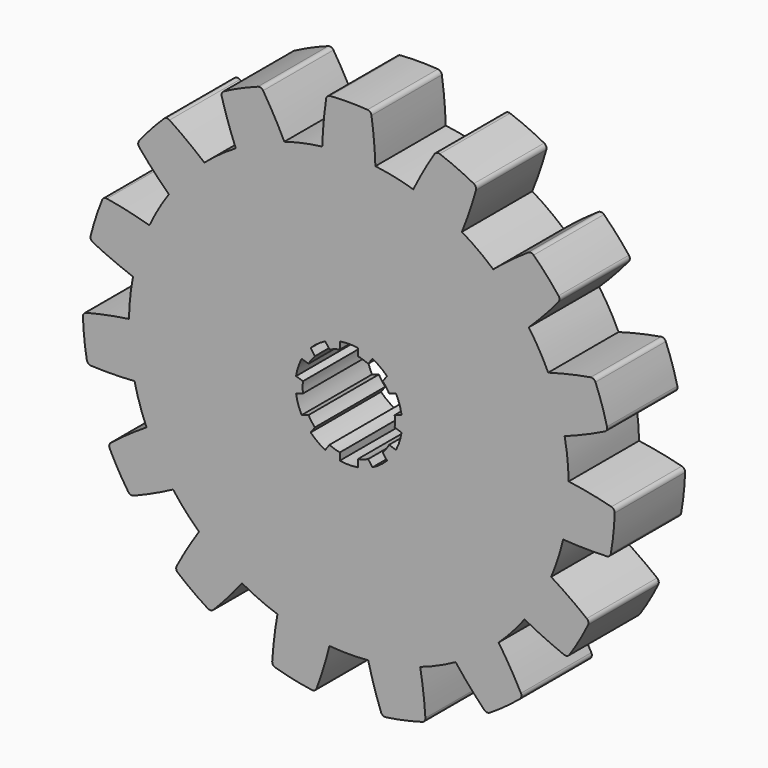
from build123d import *

# Parameters (mm, degrees)
F1_DEPTH = 20
F2_DEPTH = 20
F3_R     = 1
F4_COUNT = 15


with BuildPart() as f1:
    # F0 (on Front) → F1 (new body)
    with BuildSketch(Plane.XZ):
        with BuildLine():
            ThreePointArc((-6.0454455831, 49.6331803102), (0, 50), (6.0454455831, 49.6331803102))
            ThreePointArc((6.0454455831, 49.6331803102), (5.6999328162, 54.9765582241), (5.0372687356, 60.2899321917))
            ThreePointArc((5.0372687356, 60.2899321917), (0, 60.5), (-5.0372687356, 60.2899321917))
            ThreePointArc((-5.0372687356, 60.2899321917), (-5.6999328162, 54.9765582241), (-6.0454455831, 49.6331803102))
        make_face()
    extrude(amount=F1_DEPTH)

    # F3
    f3_edges = [f1.edges().sort_by_distance(p)[0] for p in [
        (-5.037269, -10, 60.289932),
        (5.037269, -10, 60.289932),
    ]]
    fillet(f3_edges, radius=F3_R)



with BuildPart() as f2:
    # F0 (on Front) → F2 (new body)
    with BuildSketch(Plane.XZ):
        with BuildLine():
            ThreePointArc((-6.0454455831, 49.6331803102), (-33.14911553, -37.4317530925), (50, 0))
            ThreePointArc((50, 0), (37.4317530925, 33.14911553), (6.0454455831, 49.6331803102))
            ThreePointArc((6.0454455831, 49.6331803102), (0, 50), (-6.0454455831, 49.6331803102))
        make_face()
        with BuildLine():
            ThreePointArc((10.4274046286, 1.2325715847), (10.4818354452, 0.6173537882), (10.5, 0))
            ThreePointArc((10.5, 0), (10.4818354452, -0.6173537882), (10.4274046286, -1.2325715847))
            Line((10.4274046286, -1.2325715847), (11.9961998639, -1.742304056))
            ThreePointArc((11.9961998639, -1.742304056), (11.5230272808, -3.7440585238), (10.729230187, -5.6416357729))
            Line((10.729230187, -5.6416357729), (9.1604349517, -5.1319033015))
            ThreePointArc((9.1604349517, -5.1319033015), (8.4946784409, -6.1717451491), (7.7114601519, -7.1262460192))
            Line((7.7114601519, -7.1262460192), (8.6810289287, -8.4607429543))
            ThreePointArc((8.6810289287, -8.4607429543), (7.1216225128, -9.8020724711), (5.3640592517, -10.8706624887))
            Line((5.3640592517, -10.8706624887), (4.3944904749, -9.5361655536))
            ThreePointArc((4.3944904749, -9.5361655536), (3.2446784409, -9.9860934211), (2.05, -10.2979366865))
            Line((2.05, -10.2979366865), (2.05, -11.947465614))
            ThreePointArc((2.05, -11.947465614), (0, -12.1160278946), (-2.05, -11.947465614))
            Line((-2.05, -11.947465614), (-2.05, -10.2979366865))
            ThreePointArc((-2.05, -10.2979366865), (-3.2446784409, -9.9860934211), (-4.3944904749, -9.5361655536))
            Line((-4.3944904749, -9.5361655536), (-5.3640592517, -10.8706624887))
            ThreePointArc((-5.3640592517, -10.8706624887), (-7.1216225128, -9.8020724711), (-8.6810289287, -8.4607429543))
            Line((-8.6810289287, -8.4607429543), (-7.7114601519, -7.1262460192))
            ThreePointArc((-7.7114601519, -7.1262460192), (-8.4946784409, -6.1717451491), (-9.1604349517, -5.1319033015))
            Line((-9.1604349517, -5.1319033015), (-10.729230187, -5.6416357729))
            ThreePointArc((-10.729230187, -5.6416357729), (-11.5230272808, -3.7440585238), (-11.9961998639, -1.742304056))
            Line((-11.9961998639, -1.742304056), (-10.4274046286, -1.2325715847))
            ThreePointArc((-10.4274046286, -1.2325715847), (-10.5, 0), (-10.4274046286, 1.2325715847))
            Line((-10.4274046286, 1.2325715847), (-11.9961998639, 1.742304056))
            ThreePointArc((-11.9961998639, 1.742304056), (-11.5230272808, 3.7440585238), (-10.729230187, 5.6416357729))
            Line((-10.729230187, 5.6416357729), (-9.1604349517, 5.1319033015))
            ThreePointArc((-9.1604349517, 5.1319033015), (-8.4946784409, 6.1717451491), (-7.7114601519, 7.1262460192))
            Line((-7.7114601519, 7.1262460192), (-8.6810289287, 8.4607429543))
            ThreePointArc((-8.6810289287, 8.4607429543), (-7.1216225128, 9.8020724711), (-5.3640592517, 10.8706624887))
            Line((-5.3640592517, 10.8706624887), (-4.3944904749, 9.5361655536))
            ThreePointArc((-4.3944904749, 9.5361655536), (-3.2446784409, 9.9860934211), (-2.05, 10.2979366865))
            Line((-2.05, 10.2979366865), (-2.05, 11.947465614))
            ThreePointArc((-2.05, 11.947465614), (0, 12.1160278946), (2.05, 11.947465614))
            Line((2.05, 11.947465614), (2.05, 10.2979366865))
            ThreePointArc((2.05, 10.2979366865), (3.2446784409, 9.9860934211), (4.3944904749, 9.5361655536))
            Line((4.3944904749, 9.5361655536), (5.3640592517, 10.8706624887))
            ThreePointArc((5.3640592517, 10.8706624887), (7.1216225128, 9.8020724711), (8.6810289287, 8.4607429543))
            Line((8.6810289287, 8.4607429543), (7.7114601519, 7.1262460192))
            ThreePointArc((7.7114601519, 7.1262460192), (8.4946784409, 6.1717451491), (9.1604349517, 5.1319033015))
            Line((9.1604349517, 5.1319033015), (10.729230187, 5.6416357729))
            ThreePointArc((10.729230187, 5.6416357729), (11.5230272808, 3.7440585238), (11.9961998639, 1.742304056))
            Line((11.9961998639, 1.742304056), (10.4274046286, 1.2325715847))
        make_face(mode=Mode.SUBTRACT)
    extrude(amount=F2_DEPTH)


with BuildPart() as f1_1:
    add(f1.part)

    add(f2.part)  # F4 merges F2
    # F4: F1 ×15 about axis
    f4_axis = Axis((0, 0, 0), (0, -1, 0))
    for i in range(1, F4_COUNT):
        add(f1.part.rotate(f4_axis, i * 360 / F4_COUNT))


solid = f1_1.part
